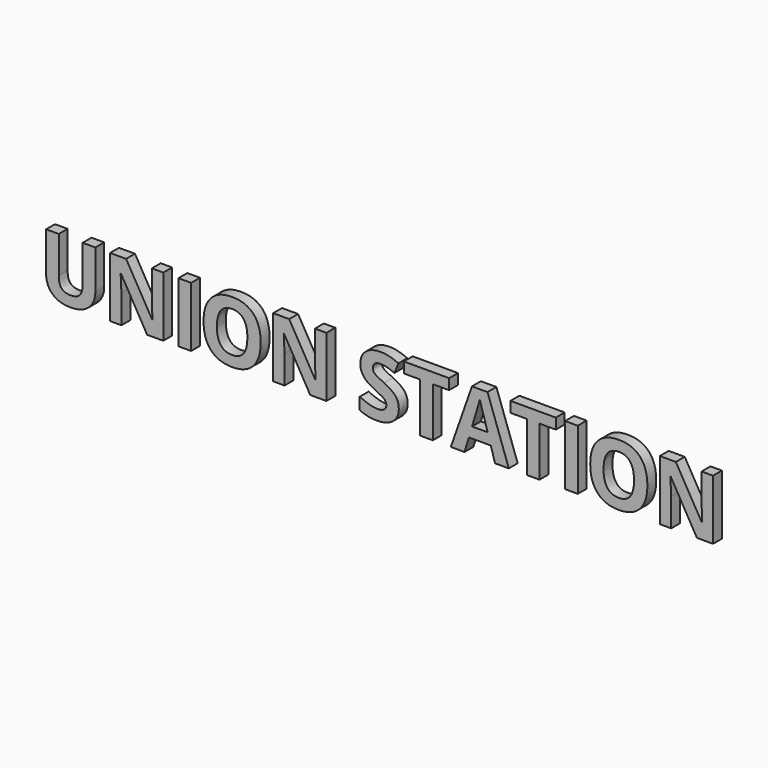
from build123d import *

# Parameters (mm, degrees)
F0_TEXT_SIZE = 288.7116538154
F1_DEPTH     = 38.1


# Not quite as in the source:
# - Text() gives the source's letters only with a copy of the font that has no kerning and outlines rounded to 1/6400 em; it was checked with that copy


with BuildPart() as f1:
    # F0 (on Front) → F1 (new body)
    with BuildSketch(Plane.XZ):
        with Locations((-1183.0314397812, -104.6434789896)):
            Text('UNION STATION', F0_TEXT_SIZE, font='Open Sans', font_style=FontStyle.BOLD, text_align=(TextAlign.LEFT, TextAlign.BOTTOM))
    extrude(amount=F1_DEPTH)


solid = f1.part
